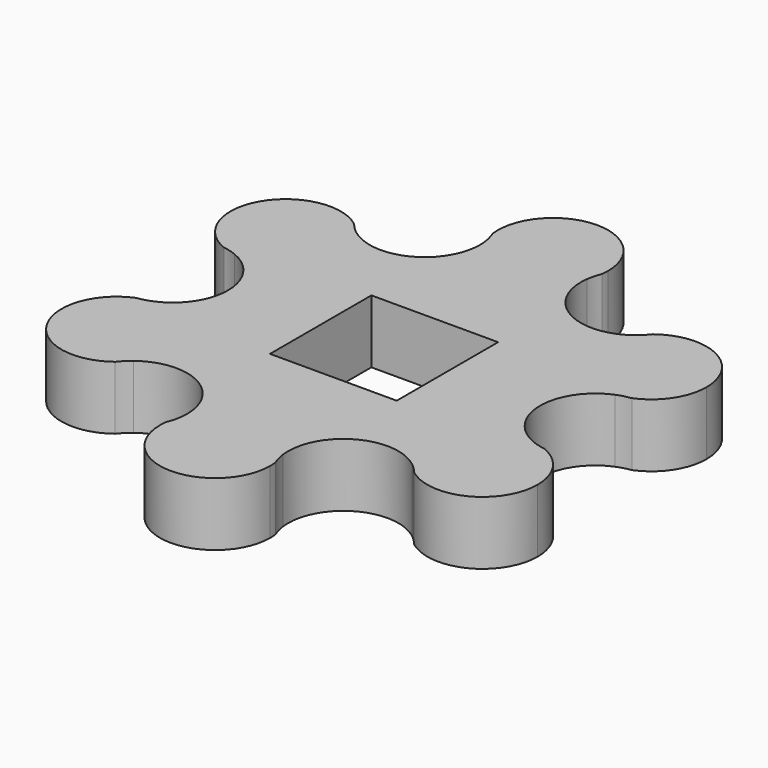
from build123d import *

# Parameters (mm, degrees)
F0_W     = 12
F0_H     = 12
F1_DEPTH = 6


with BuildPart() as f1:
    # F0 (on Top) → F1 (new body)
    with BuildSketch(Plane.XY):
        with BuildLine():
            ThreePointArc((18.0019915499, 4.8236190979), (18.6486934227, 5.0431448029), (19.3185165258, 5.1763809021))
            ThreePointArc((19.3185165258, 5.1763809021), (17.3205080757, 10), (14.1421356237, 14.1421356237))
            ThreePointArc((14.1421356237, 14.1421356237), (13.6918382257, 13.62866985), (13.178372452, 13.178372452))
            ThreePointArc((13.178372452, 13.178372452), (12.7989481428, 7.3894761556), (18.0019915499, 4.8236190979))
        make_face()
        with BuildLine():
            ThreePointArc((14.1421356237, 14.1421356237), (17.3205080757, 10), (19.3185165258, 5.1763809021))
            ThreePointArc((19.3185165258, 5.1763809021), (21.6616505733, 7.0993413189), (22.5415557645, 10))
            ThreePointArc((22.5415557645, 10), (19.6297184195, 14.6826153543), (14.1421356237, 14.1421356237))
        make_face()
        with BuildLine():
            ThreePointArc((22.5415557645, -10), (21.6616505733, -7.0993413189), (19.3185165258, -5.1763809021))
            ThreePointArc((19.3185165258, -5.1763809021), (17.3205080757, -10), (14.1421356237, -14.1421356237))
            ThreePointArc((14.1421356237, -14.1421356237), (19.6297184195, -14.6826153543), (22.5415557645, -10))
        make_face()
        with BuildLine():
            ThreePointArc((14.1421356237, -14.1421356237), (17.3205080757, -10), (19.3185165258, -5.1763809021))
            ThreePointArc((19.3185165258, -5.1763809021), (18.6486934227, -5.0431448029), (18.0019915499, -4.8236190979))
            ThreePointArc((18.0019915499, -4.8236190979), (12.7989481428, -7.3894761556), (13.178372452, -13.178372452))
            ThreePointArc((13.178372452, -13.178372452), (13.6918382257, -13.62866985), (14.1421356237, -14.1421356237))
        make_face()
        with BuildLine():
            ThreePointArc((18.0019915499, -4.8236190979), (14.7789523112, 0), (18.0019915499, 4.8236190979))
            ThreePointArc((18.0019915499, 4.8236190979), (12.7989481428, 7.3894761556), (13.178372452, 13.178372452))
            ThreePointArc((13.178372452, 13.178372452), (7.3894761556, 12.7989481428), (4.8236190979, 18.0019915499))
            ThreePointArc((4.8236190979, 18.0019915499), (0, 14.7789523112), (-4.8236190979, 18.0019915499))
            ThreePointArc((-4.8236190979, 18.0019915499), (-4.7901309751, 17.6619809324), (-4.7789523112, 17.3205080757))
            ThreePointArc((-4.7789523112, 17.3205080757), (-7.6907896561, 12.6378927214), (-13.178372452, 13.178372452))
            ThreePointArc((-13.178372452, 13.178372452), (-12.3765407116, 11.6782507774), (-12.0994603869, 10))
            ThreePointArc((-12.0994603869, 10), (-13.8780321316, 6.0746085108), (-18.0019915499, 4.8236190979))
            ThreePointArc((-18.0019915499, 4.8236190979), (-15.6588575024, 2.9006586811), (-14.7789523112, 0))
            ThreePointArc((-14.7789523112, 0), (-15.6588575024, -2.9006586811), (-18.0019915499, -4.8236190979))
            ThreePointArc((-18.0019915499, -4.8236190979), (-13.8780321316, -6.0746085108), (-12.0994603869, -10))
            ThreePointArc((-12.0994603869, -10), (-12.3765407116, -11.6782507774), (-13.178372452, -13.178372452))
            ThreePointArc((-13.178372452, -13.178372452), (-7.6907896561, -12.6378927214), (-4.7789523112, -17.3205080757))
            ThreePointArc((-4.7789523112, -17.3205080757), (-4.7901309751, -17.6619809324), (-4.8236190979, -18.0019915499))
            ThreePointArc((-4.8236190979, -18.0019915499), (0, -14.7789523112), (4.8236190979, -18.0019915499))
            ThreePointArc((4.8236190979, -18.0019915499), (7.3894761556, -12.7989481428), (13.178372452, -13.178372452))
            ThreePointArc((13.178372452, -13.178372452), (12.7989481428, -7.3894761556), (18.0019915499, -4.8236190979))
        make_face()
        Rectangle(F0_W, F0_H, mode=Mode.SUBTRACT)
        with BuildLine():
            ThreePointArc((4.8236190979, 18.0019915499), (4.9568551971, 18.6718146529), (5.1763809021, 19.3185165258))
            ThreePointArc((5.1763809021, 19.3185165258), (0, 20), (-5.1763809021, 19.3185165258))
            ThreePointArc((-5.1763809021, 19.3185165258), (-4.9568551971, 18.6718146529), (-4.8236190979, 18.0019915499))
            ThreePointArc((-4.8236190979, 18.0019915499), (0, 14.7789523112), (4.8236190979, 18.0019915499))
        make_face()
        with BuildLine():
            ThreePointArc((-5.1763809021, 19.3185165258), (0, 20), (5.1763809021, 19.3185165258))
            ThreePointArc((5.1763809021, 19.3185165258), (5.2098690249, 19.6585271433), (5.2210476888, 20))
            ThreePointArc((5.2210476888, 20), (-0.3414728567, 25.2098690249), (-5.1763809021, 19.3185165258))
        make_face()
        with BuildLine():
            ThreePointArc((5.2210476888, -20), (5.2098690249, -19.6585271433), (5.1763809021, -19.3185165258))
            ThreePointArc((5.1763809021, -19.3185165258), (0, -20), (-5.1763809021, -19.3185165258))
            ThreePointArc((-5.1763809021, -19.3185165258), (-0.3414728567, -25.2098690249), (5.2210476888, -20))
        make_face()
        with BuildLine():
            ThreePointArc((-5.1763809021, -19.3185165258), (0, -20), (5.1763809021, -19.3185165258))
            ThreePointArc((5.1763809021, -19.3185165258), (4.9568551971, -18.6718146529), (4.8236190979, -18.0019915499))
            ThreePointArc((4.8236190979, -18.0019915499), (0, -14.7789523112), (-4.8236190979, -18.0019915499))
            ThreePointArc((-4.8236190979, -18.0019915499), (-4.9568551971, -18.6718146529), (-5.1763809021, -19.3185165258))
        make_face()
        with BuildLine():
            ThreePointArc((-13.178372452, 13.178372452), (-13.6918382257, 13.62866985), (-14.1421356237, 14.1421356237))
            ThreePointArc((-14.1421356237, 14.1421356237), (-17.3205080757, 10), (-19.3185165258, 5.1763809021))
            ThreePointArc((-19.3185165258, 5.1763809021), (-18.6486934227, 5.0431448029), (-18.0019915499, 4.8236190979))
            ThreePointArc((-18.0019915499, 4.8236190979), (-13.8780321316, 6.0746085108), (-12.0994603869, 10))
            ThreePointArc((-12.0994603869, 10), (-12.3765407116, 11.6782507774), (-13.178372452, 13.178372452))
        make_face()
        with BuildLine():
            ThreePointArc((-19.3185165258, 5.1763809021), (-17.3205080757, 10), (-14.1421356237, 14.1421356237))
            ThreePointArc((-14.1421356237, 14.1421356237), (-21.8420680086, 12.6105238444), (-19.3185165258, 5.1763809021))
        make_face()
        with BuildLine():
            ThreePointArc((-19.3185165258, -5.1763809021), (-21.8420680086, -12.6105238444), (-14.1421356237, -14.1421356237))
            ThreePointArc((-14.1421356237, -14.1421356237), (-17.3205080757, -10), (-19.3185165258, -5.1763809021))
        make_face()
        with BuildLine():
            ThreePointArc((-19.3185165258, -5.1763809021), (-17.3205080757, -10), (-14.1421356237, -14.1421356237))
            ThreePointArc((-14.1421356237, -14.1421356237), (-13.6918382257, -13.62866985), (-13.178372452, -13.178372452))
            ThreePointArc((-13.178372452, -13.178372452), (-12.3765407116, -11.6782507774), (-12.0994603869, -10))
            ThreePointArc((-12.0994603869, -10), (-13.8780321316, -6.0746085108), (-18.0019915499, -4.8236190979))
            ThreePointArc((-18.0019915499, -4.8236190979), (-18.6486934227, -5.0431448029), (-19.3185165258, -5.1763809021))
        make_face()
    extrude(amount=F1_DEPTH)


solid = f1.part
